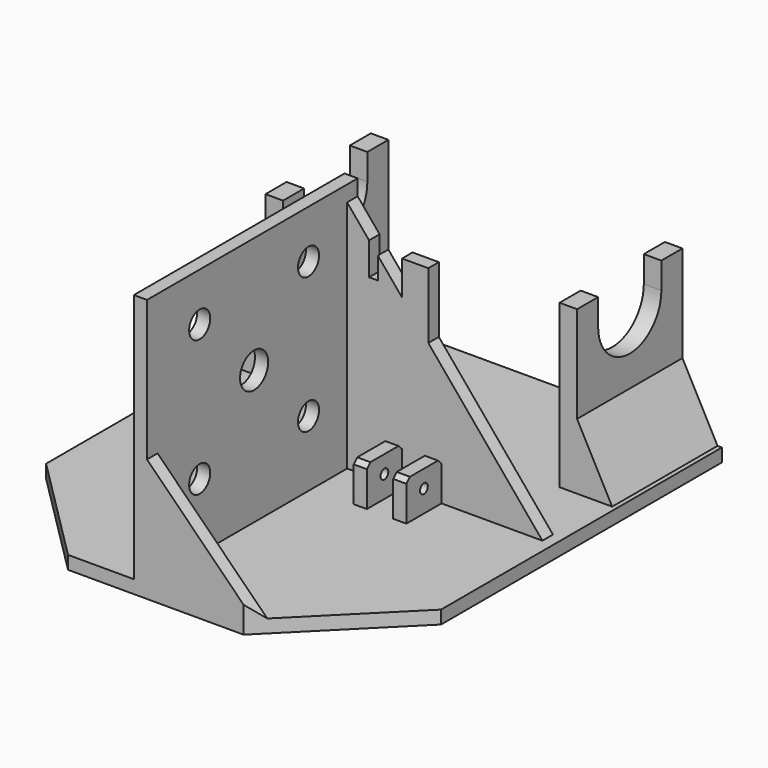
from build123d import *

# Parameters (mm, degrees)
F0_W      = 40
F0_H      = 60
F0_W_2    = 50
F0_W_3    = 3
F0_H_2    = 10
F1_DEPTH  = 3
F0_W_4    = 4
F0_H_3    = 30
F2_DEPTH  = 40
F3_DEPTH  = 12
F4_SIZE   = 1
F5_R      = 1.1
F6_DEPTH  = 13
F7_W      = 60
F7_H      = 60
F7_R      = 3
F7_R_2    = 4
F8_DEPTH  = 3
F10_DEPTH = 3
F12_DEPTH = 100
F14_DEPTH = 3
F15_SIZE  = 24.99999
F17_DEPTH = 30


# Not quite as in the source:
# - a fillet or chamfer is up to 0.001 mm smaller than in the source, because OpenCascade refuses the exact size
# - a feature names something its author has since deleted; it is built from what else it names


with BuildPart() as f1:
    # F0 (on Top) → F1 (new body)
    with BuildSketch(Plane.XY):
        with Locations((-20, -30)):
            Rectangle(F0_W, F0_H)
        with Locations((25, -30)):
            Rectangle(F0_W_2, F0_H)
        with Locations((14, -8)):
            Rectangle(F0_W_3, F0_H_2, mode=Mode.SUBTRACT)
        with Locations((23, -8)):
            Rectangle(F0_W_3, F0_H_2, mode=Mode.SUBTRACT)
        Polygon((0, 45), (0, 0), (50, 0), (50, 45), (41, 45), (41, 15), (37, 15), (37, 45), align=None)
        Polygon((-40, 0), (0, 0), (0, 45), (-26, 45), (-26, 15), (-30, 15), (-30, 45), (-40, 45), align=None)
    extrude(amount=F1_DEPTH)

    # F0 (on Top) → F2 (join)
    with BuildSketch(Plane.XY):
        with Locations((-28, 30)):
            Rectangle(F0_W_4, F0_H_3)
        with Locations((39, 30)):
            Rectangle(F0_W_4, F0_H_3)
    extrude(amount=F2_DEPTH)

    # F0 (on Top) → F3 (join)
    with BuildSketch(Plane.XY):
        with Locations((23, -8)):
            Rectangle(F0_W_3, F0_H_2)
        with Locations((14, -8)):
            Rectangle(F0_W_3, F0_H_2)
    extrude(amount=F3_DEPTH)

    # F4
    f4_edges = [f1.edges().sort_by_distance(p)[0] for p in [
        (14, -3, 12),
        (23, -3, 12),
        (23, -13, 12),
        (14, -13, 12),
    ]]
    chamfer(f4_edges, length=F4_SIZE)

    # F5 (on face) → F6 (cut)
    with BuildSketch(Plane.YZ.offset(24.5)):
        with Locations((-8, 8)):
            Circle(F5_R)
    extrude(amount=-F6_DEPTH, mode=Mode.SUBTRACT)

    # F7 (on Right) → F8 (join)
    with BuildSketch(Plane.YZ):
        with Locations((-30, 30)):
            Rectangle(F7_W, F7_H)
        with Locations((-45, 18)):
            Circle(F7_R, mode=Mode.SUBTRACT)
        with Locations((-14, 18)):
            Circle(F7_R, mode=Mode.SUBTRACT)
        with Locations((-45, 49)):
            Circle(F7_R, mode=Mode.SUBTRACT)
        with Locations((-29.5, 33.5)):
            Circle(F7_R_2, mode=Mode.SUBTRACT)
        with Locations((-14, 49)):
            Circle(F7_R, mode=Mode.SUBTRACT)
    extrude(amount=F8_DEPTH)

    # F9 (on Front) → F10 (join)
    with BuildSketch(Plane.XZ):
        Polygon((0, 60), (0, 0), (50, 0), (21.5, 34.2), (15.5, 41.4), (10, 48), (10, 43), (8, 43), (8, 50.4), align=None)
        Polygon((15.5, 41.4), (21.5, 34.2), (21.5, 49.2), (15.5, 49.2), align=None)
    extrude(amount=F10_DEPTH)

    # F11 (on face) → F12 (cut)
    with BuildSketch(Plane.YZ.offset(41)):
        with BuildLine():
            Line((21, 40), (23.2917960675, 40))
            ThreePointArc((23.2917960675, 40), (30, 43), (36.7082039325, 40))
            Line((36.7082039325, 40), (39, 40))
            Line((39, 40), (39, 47))
            Line((39, 47), (21, 47))
            Line((21, 47), (21, 40))
        make_face()
        with BuildLine():
            ThreePointArc((23.2917960675, 40), (21.5924487693, 37.211398808), (21, 34))
            ThreePointArc((21, 34), (30, 25), (39, 34))
            ThreePointArc((39, 34), (38.4075512307, 37.211398808), (36.7082039325, 40))
            Line((36.7082039325, 40), (23.2917960675, 40))
        make_face()
        with BuildLine():
            Line((21, 40), (21, 34))
            ThreePointArc((21, 34), (21.5924487693, 37.211398808), (23.2917960675, 40))
            Line((23.2917960675, 40), (21, 40))
        make_face()
        with BuildLine():
            ThreePointArc((36.7082039325, 40), (38.4075512307, 37.211398808), (39, 34))
            Line((39, 34), (39, 40))
            Line((39, 40), (36.7082039325, 40))
        make_face()
    extrude(amount=-F12_DEPTH, mode=Mode.SUBTRACT)

    # F13 (on face) → F14 (join)
    with BuildSketch(Plane.XZ.offset(60)):
        Polygon((3, 28), (3, 3), (28, 3), align=None)
    extrude(amount=-F14_DEPTH)

    # F15 (size 25 in the source; OpenCascade refuses exactly that, so slightly less here)
    f15_edges = [f1.edges().sort_by_distance(p)[0] for p in [
        (50, -60, 1.5),
        (-40, -60, 1.5),
    ]]
    chamfer(f15_edges, length=F15_SIZE)

    # F16 (on face) → F17 (join)
    with BuildSketch(Plane(origin=(0, 45, 0), x_dir=(-1, 0, 0), z_dir=(0, 1, 0))):
        Polygon((30, 3), (38, 3), (30, 18), align=None)
        Polygon((-49, 3), (-41, 3), (-41, 18), align=None)
    extrude(amount=-F17_DEPTH)


solid = f1.part
